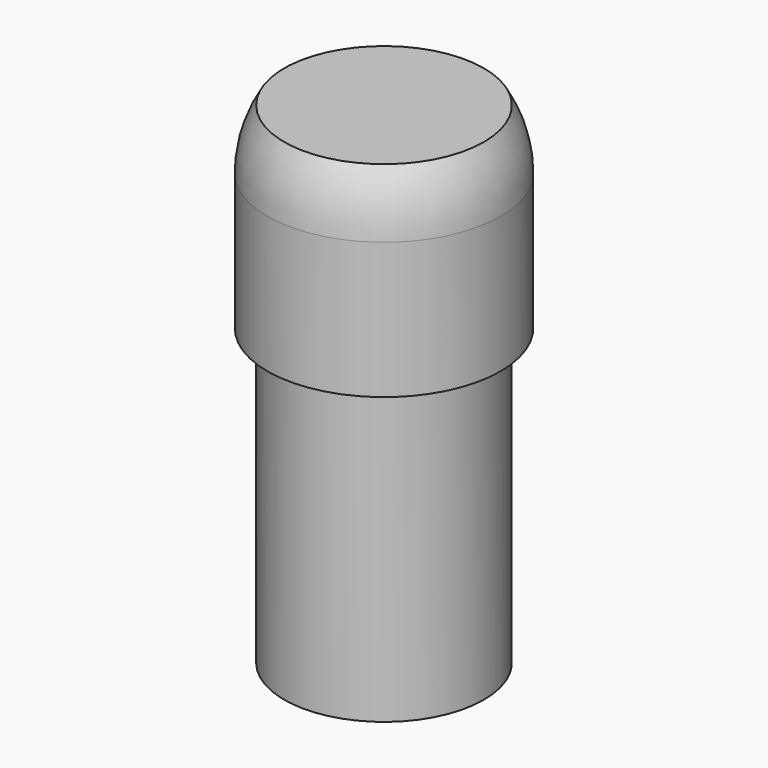
from build123d import *

# Parameters (mm, degrees)
F0_R     = 25.8318
F1_DEPTH = 76.2
F2_R     = 30.1498
F2_R_2   = 25.8318
F3_DEPTH = 50.8
F4_DEPTH = 50.8


# Not quite as in the source:
# - a fillet or chamfer that OpenCascade refuses, or shapes differently, is made with other operations: its cross-section is extruded or revolved along the edge and cut away or added


with BuildPart() as f1:
    # F0 (on Top) → F1 (new body)
    with BuildSketch(Plane.XY):
        Circle(F0_R)
    extrude(amount=F1_DEPTH)


with BuildPart() as f3:
    # F2 (on face) → F3 (new body)
    with BuildSketch(Plane.XY.offset(76.2)):
        Circle(F2_R)
        Circle(F2_R_2, mode=Mode.SUBTRACT)
    extrude(amount=F3_DEPTH)

    # F5: fillet of radius 30.1244 on 1 edges, made by hand

    # F5_s1 → F5_t2 (revolve, cut)
    with BuildSketch(Plane.XZ):
        with BuildLine():
            ThreePointArc((30.1498, 111.4594339099), (29.0502323985, 119.5240839085), (25.8318, 127))
            Line((25.8318, 127), (30.1498, 127))
            Line((30.1498, 127), (30.1498, 111.4594339099))
        make_face()
    revolve(axis=Axis((0, 0, 127), (0, 0, 1)), mode=Mode.SUBTRACT)


with BuildPart() as f4:
    # F4 (new): a face of the model
    f4_faces = [f1.part.faces().sort_by_distance(p)[0] for p in [
        (0, 0, 76.2),
    ]]
    extrude(f4_faces, amount=F4_DEPTH)


solid = Compound([f1.part, f3.part, f4.part])
